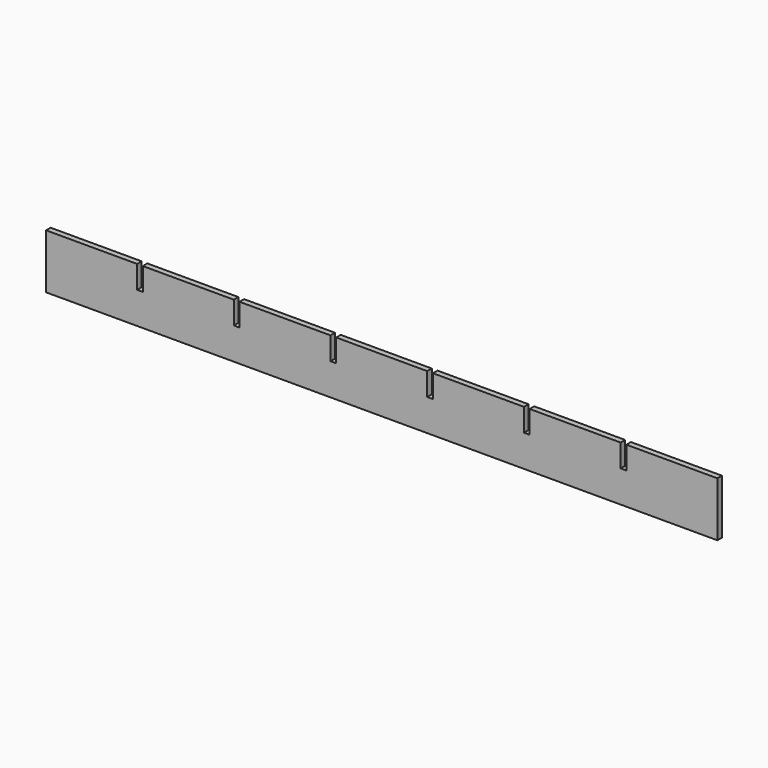
from build123d import *

# Parameters (mm, degrees)
F1_DEPTH = 3.175


# Not quite as in the source:
# - a length typed as a fraction of an inch, garbled in the dataset ("3 / 203.2 mm" for 3/8 in), is restored


with BuildPart() as f1:
    # F0 (on Front) → F1 (new body)
    with BuildSketch(Plane.XZ):
        Polygon((-230.5319600344, -49.02207428), (-281.3319600344, -49.02207428), (-281.3319600344, -79.50207428), (93.3180399656, -79.50207428), (93.3180399656, -61.72207428), (93.3180399656, -49.02207428), (42.5180399656, -49.02207428), (42.5180399656, -61.72207428), (39.3430399656, -61.72207428), (39.3430399656, -49.02207428), (-11.4569600344, -49.02207428), (-11.4569600344, -61.72207428), (-14.6319600344, -61.72207428), (-14.6319600344, -49.02207428), (-65.4319600344, -49.02207428), (-65.4319600344, -61.72207428), (-68.6069600344, -61.72207428), (-68.6069600344, -49.02207428), (-119.4069600344, -49.02207428), (-119.4069600344, -61.72207428), (-122.5819600344, -61.72207428), (-122.5819600344, -49.02207428), (-173.3819600344, -49.02207428), (-173.3819600344, -61.72207428), (-176.5569600344, -61.72207428), (-176.5569600344, -49.02207428), (-227.3569600344, -49.02207428), (-227.3569600344, -61.72207428), (-230.5319600344, -61.72207428), align=None)
    extrude(amount=F1_DEPTH)


solid = f1.part
